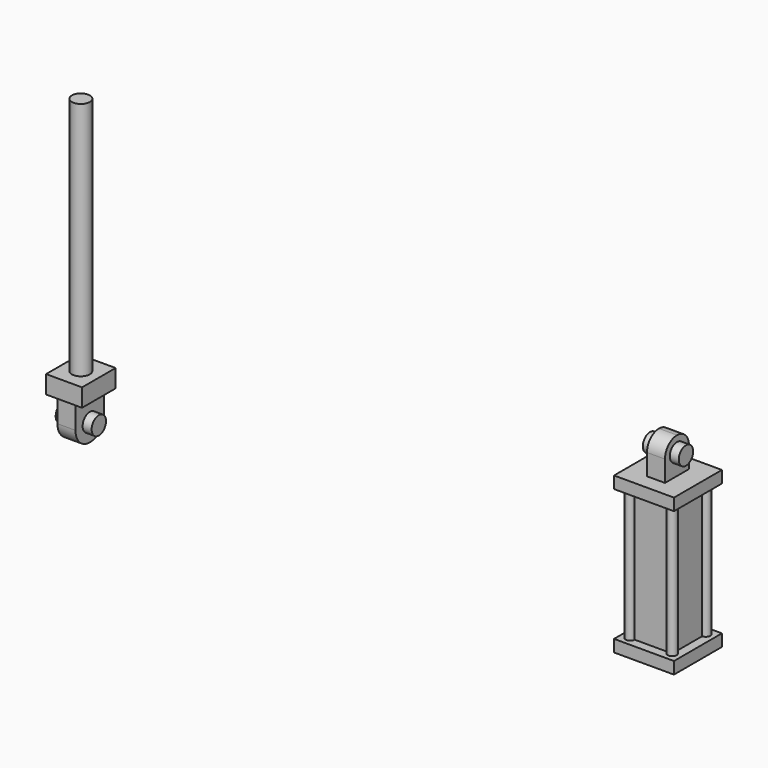
from build123d import *

# Parameters (mm, degrees)
F0_W           = 2.54
F0_H           = 2.54
F1_DEPTH       = 0.508
F3_R           = 0.1905
F2_W           = 1.778
F2_H           = 1.778
F4_DEPTH       = 5.588
F5_W           = 2.54
F5_H           = 2.54
F6_DEPTH       = 0.508
F7_W           = 0.762
F7_H           = 1.27
F8_DEPTH       = 1.524
F9_R           = 0.63499
F10_R          = 0.381
F11_DEPTH      = 0.254
F12_W          = 1.524
F12_H          = 1.778
F13_DEPTH      = 0.762
F14_R          = 0.381
F15_DEPTH      = 10.16
F16_W          = 0.762
F16_H          = 1.524
F17_DEPTH      = 1.778
F18_R          = 0.76199
F19_R          = 0.381
F20_DEPTH      = 0.381
F20_DEPTH_BACK = 1.143
F21_R          = 0.381
F22_DEPTH      = 0.381
F22_DEPTH_BACK = 1.143


# Not quite as in the source:
# - a fillet or chamfer is up to 0.001 mm smaller than in the source, because OpenCascade refuses the exact size
# - a feature names something its author has since deleted; it is built from what else it names


with BuildPart() as f1:
    # F0 (on Top) → F1 (new body)
    with BuildSketch(Plane.XY):
        with Locations((-1.27, 1.27)):
            Rectangle(F0_W, F0_H)
    extrude(amount=F1_DEPTH)

    # F3 (on face) + F2 (on face) → F4 (join)
    with BuildSketch(Plane.XY.offset(0.508)):
        with Locations((-2.159, 0.381)):
            Circle(F3_R)
        with Locations((-0.381, 0.381)):
            Circle(F3_R)
        with Locations((-0.381, 2.159)):
            Circle(F3_R)
        with Locations((-2.159, 2.159)):
            Circle(F3_R)
    with BuildSketch(Plane.XY.offset(0.508)):
        with Locations((-1.27, 1.27)):
            Rectangle(F2_W, F2_H)
    extrude(amount=F4_DEPTH)

    # F5 (on face) → F6 (join)
    with BuildSketch(Plane.XY.offset(6.096)):
        with Locations((-1.27, 1.27)):
            Rectangle(F5_W, F5_H)
    extrude(amount=F6_DEPTH)

    # F7 (on face) → F8 (join)
    with BuildSketch(Plane.XY.offset(6.604)):
        with Locations((-1.27, 1.27)):
            Rectangle(F7_W, F7_H)
    extrude(amount=F8_DEPTH)

    # F9 (radius 0.635 in the source; OpenCascade refuses exactly that, so slightly less here)
    f9_edges = [f1.edges().sort_by_distance(p)[0] for p in [
        (-1.27, 0.635, 8.128),
        (-1.27, 1.905, 8.128),
    ]]
    fillet(f9_edges, radius=F9_R)

    # F10 (on face) → F11 (cut)
    with BuildSketch(Plane(origin=(0, 0, 0), x_dir=(1, 0, 0), z_dir=(0, 0, -1))):
        with Locations((-1.27, -1.27)):
            Circle(F10_R)
    extrude(amount=-F11_DEPTH, mode=Mode.SUBTRACT)

    # F19 (on face) → F20 (join, two sides)
    with BuildSketch(Plane.YZ.offset(-0.889)) as f20_sk:
        with Locations((1.27, 7.493)):
            Circle(F19_R)
    extrude(amount=F20_DEPTH)
    extrude(f20_sk.sketch, amount=-F20_DEPTH_BACK)


with BuildPart() as f13:
    # F12 (on Top) → F13 (new body)
    with BuildSketch(Plane.XY):
        with Locations((-28.0019982215, 3.5851696832)):
            Rectangle(F12_W, F12_H)
    extrude(amount=F13_DEPTH)

    # F14 (on face) → F15 (join)
    with BuildSketch(Plane.XY.offset(0.762)):
        with Locations((-28.0019982215, 3.5851696832)):
            Circle(F14_R)
    extrude(amount=F15_DEPTH)

    # F16 (on face) → F17 (join)
    with BuildSketch(Plane(origin=(0, 0, 0), x_dir=(1, 0, 0), z_dir=(0, 0, -1))):
        with Locations((-28.0019982215, -3.5851696832)):
            Rectangle(F16_W, F16_H)
    extrude(amount=F17_DEPTH)

    # F18 (radius 0.762 in the source; OpenCascade refuses exactly that, so slightly less here)
    f18_edges = [f13.edges().sort_by_distance(p)[0] for p in [
        (-28.001998, 2.82317, -1.778),
        (-28.001998, 4.34717, -1.778),
    ]]
    fillet(f18_edges, radius=F18_R)

    # F21 (on face) → F22 (join, two sides)
    with BuildSketch(Plane.YZ.offset(-27.6209982215)) as f22_sk:
        with Locations((3.5851696832, -1.016)):
            Circle(F21_R)
    extrude(amount=F22_DEPTH)
    extrude(f22_sk.sketch, amount=-F22_DEPTH_BACK)


solid = Compound([f1.part, f13.part])
